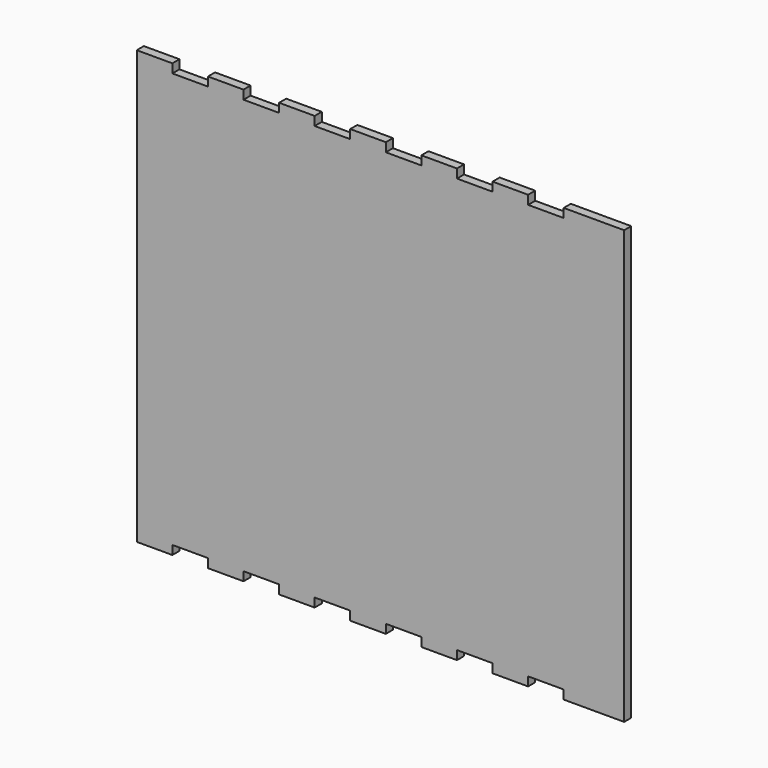
from build123d import *

# Parameters (mm, degrees)
F1_DEPTH = 3


# Not quite as in the source:
# - ends of sketch curves that miss each other by under 0.0002 mm in the source are joined


with BuildPart() as f1:
    # F0 (on Front) → F1 (new body)
    with BuildSketch(Plane.XZ):
        Polygon((-66, 73), (-78, 73), (-78, -73), (-66, -73), (-66, -70), (-54, -70), (-54, -73), (-42, -73), (-42, -70), (-30, -70), (-30, -73), (-18, -73), (-17.9999983907, -70), (-5.9999983907, -70), (-5.9999983907, -73), (6.0000016093, -73), (6.0000016093, -70), (18.0000016093, -70), (18.0000016093, -73), (30.0000016093, -73), (30.0000016093, -70), (42.0000016093, -70), (42.0000016093, -73), (54.0000016093, -73), (54.0000016093, -70), (66.0000016093, -70), (66.0000016093, -73), (86.38356, -73), (86.38356, 73), (66, 73), (66, 70), (54, 70), (54, 73), (42, 73), (42, 70), (30, 70), (30, 73), (18, 73), (18, 70), (6, 70), (6, 73), (-6, 73), (-6, 70), (-18, 70), (-18, 73), (-30, 73), (-30, 70), (-42, 70), (-42, 73), (-54, 73), (-54, 70), (-66, 70), align=None)
    extrude(amount=F1_DEPTH)


solid = f1.part
